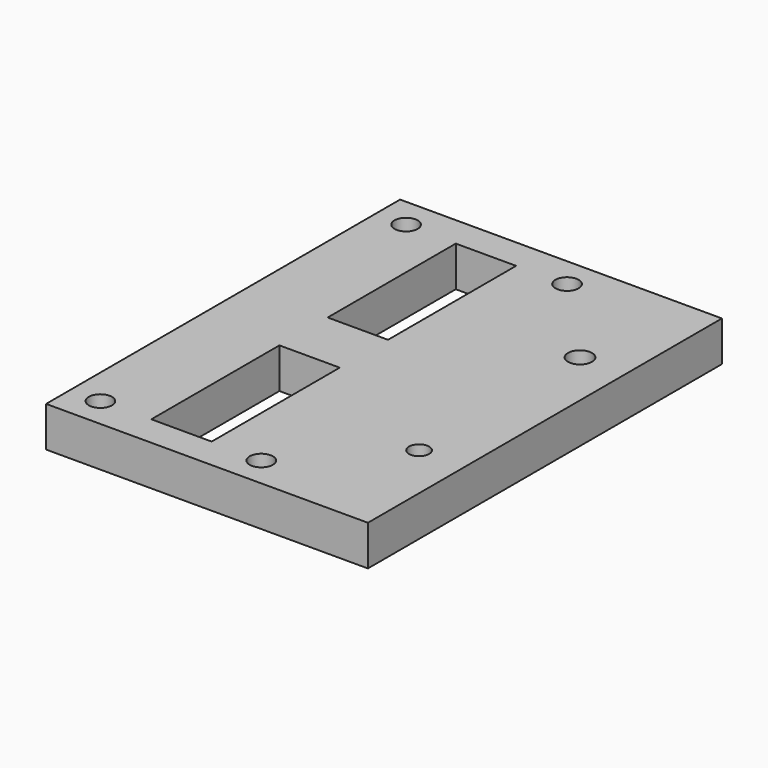
from build123d import *

# Parameters (mm, degrees)
F0_W     = 34.925
F0_H     = 69.85
F0_R     = 1.8288
F0_W_2   = 9.525
F0_H_2   = 25.273
F0_W_3   = 15.875
F0_R_2   = 1.5875
F1_DEPTH = 6.35
F2_D     = 3.6576
F3_D     = 3.7973


# Not quite as in the source:
# - a feature names something its author has since deleted; it is built from what else it names


with BuildPart() as f1:
    # F0 (on Top) → F1 (new body)
    with BuildSketch(Plane.XY):
        with Locations((-87.3125, 0)):
            Rectangle(F0_W, F0_H)
        with Locations((-100.0125, -30.1625)):
            Circle(F0_R, mode=Mode.SUBTRACT)
        with Locations((-87.3125, -17.399)):
            Rectangle(F0_W_2, F0_H_2, mode=Mode.SUBTRACT)
        with Locations((-74.6125, -30.1625)):
            Circle(F0_R, mode=Mode.SUBTRACT)
        with Locations((-87.3125, 17.399)):
            Rectangle(F0_W_2, F0_H_2, mode=Mode.SUBTRACT)
        with Locations((-100.0125, 30.1625)):
            Circle(F0_R, mode=Mode.SUBTRACT)
        with Locations((-74.6125, 30.1625)):
            Circle(F0_R, mode=Mode.SUBTRACT)
        with Locations((-61.9125, 0)):
            Rectangle(F0_W_3, F0_H)
        with Locations((-61.1378, -15.875)):
            Circle(F0_R_2, mode=Mode.SUBTRACT)
        with Locations((-61.1378, 15.875)):
            Circle(F0_R_2, mode=Mode.SUBTRACT)
        with Locations((-100.0125, -30.1625)):
            Circle(F0_R)
        with Locations((-100.0125, 30.1625)):
            Circle(F0_R)
        with Locations((-74.6125, 30.1625)):
            Circle(F0_R)
        with Locations((-74.6125, -30.1625)):
            Circle(F0_R)
        with Locations((-61.1378, 15.875)):
            Circle(F0_R_2)
    extrude(amount=F1_DEPTH)

    # F2 (through all)
    with Locations(Plane(origin=(0, 0, 0), x_dir=(1, 0, 0), z_dir=(0, 0, -1))):
        with Locations((-100.0125, -30.1625), (-74.6125, -30.1625), (-74.6125, 30.1625), (-100.0125, 30.1625)):
            Hole(F2_D / 2)

    # F3 (through all)
    with Locations(Plane(origin=(0, 0, 0), x_dir=(1, 0, 0), z_dir=(0, 0, -1))):
        with Locations((-61.1378, -15.875)):
            Hole(F3_D / 2)


solid = f1.part
